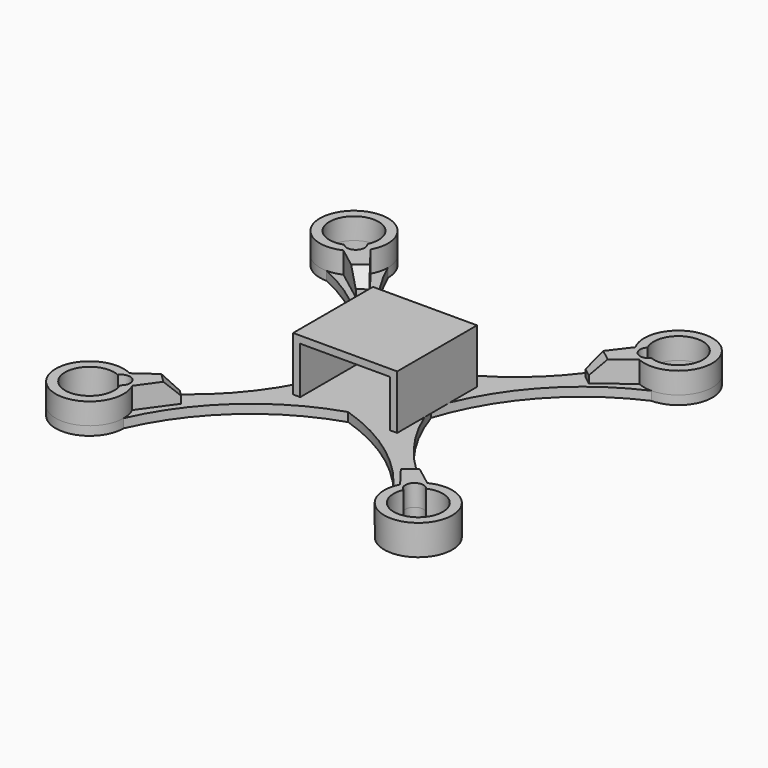
from build123d import *
from build123d import SkipClean  # not in build123d's __all__

# Parameters (mm, degrees)
F0_R     = 3.45
F1_DEPTH = 1.25
F2_R     = 1.27
F3_DEPTH = 15.24
F5_DEPTH = 7
F6_R     = 1.5
F7_DEPTH = 1.25
F9_DEPTH = 3
F10_SIZE = 2


# Not quite as in the source:
# - a feature of the source that left no trace in its solid (it failed there, or was rolled back) is left out


with BuildPart() as f1:
    # F0 (on Top) → F1 (new body)
    with BuildSketch(Plane.XY):
        with BuildLine():
            ThreePointArc((0, 6.477), (-10.7423411653, 12.8214445823), (-17.975, 22.987))
            ThreePointArc((-17.975, 22.987), (-26.1154007446, 26.3744330736), (-22.7811582525, 18.2121016594))
            ThreePointArc((-22.7811582525, 18.2121016594), (-12.6900771407, 10.8419183213), (-6.477, 0))
            ThreePointArc((-6.477, 0), (-12.7950799481, -10.8797937043), (-23.0188417475, -18.2121016594))
            ThreePointArc((-23.0188417475, -18.2121016594), (-26.4374330736, -26.3524007446), (-18.275, -22.987))
            ThreePointArc((-18.275, -22.987), (-10.9098200432, -12.770210249), (0, -6.477))
            ThreePointArc((0, -6.477), (10.9098200432, -12.770210249), (18.275, -22.987))
            ThreePointArc((18.275, -22.987), (26.4374330736, -26.3524007446), (23.0188417475, -18.2121016594))
            ThreePointArc((23.0188417475, -18.2121016594), (12.7950799481, -10.8797937043), (6.477, 0))
            ThreePointArc((6.477, 0), (12.6900771407, 10.8419183213), (22.7811582525, 18.2121016594))
            ThreePointArc((22.7811582525, 18.2121016594), (26.1154007446, 26.3744330736), (17.975, 22.987))
            ThreePointArc((17.975, 22.987), (10.7423411653, 12.8214445823), (0, 6.477))
        make_face()
        with Locations((-23.05, -22.987)):
            Circle(F0_R, mode=Mode.SUBTRACT)
        with Locations((23.05, -22.987)):
            Circle(F0_R, mode=Mode.SUBTRACT)
        with Locations((-22.75, 22.987)):
            Circle(F0_R, mode=Mode.SUBTRACT)
        with Locations((22.75, 22.987)):
            Circle(F0_R, mode=Mode.SUBTRACT)
    extrude(amount=F1_DEPTH)

    # F2 (on face) → F3 (cut)
    with BuildSketch(Plane.XY.offset(1.25)):
        with Locations((-20.5791849834, 20.5791849834)):
            Circle(F2_R)
        with Locations((20.5791849834, 20.5791849834)):
            Circle(F2_R)
        with Locations((20.5791849834, -20.5791849834)):
            Circle(F2_R)
        with Locations((-20.5791849834, -20.5791849834)):
            Circle(F2_R)
    extrude(amount=-F3_DEPTH, mode=Mode.SUBTRACT)

    # F4 (on Front) → F5 (join, symmetric)
    with BuildSketch(Plane.XZ):
        Polygon((-6.3, 1.25), (-6.3, 7.85), (6.3, 7.85), (6.3, 1.25), (7.3, 1.25), (7.3, 8.85), (-7.3, 8.85), (-7.3, 1.25), align=None)
    extrude(amount=F5_DEPTH, both=True)

    # F6 (on face) → F7 (cut, through all)
    with BuildSketch(Plane.XY.offset(1.25)):
        with Locations((0, 6.477)):
            Circle(F6_R)
    extrude(amount=-F7_DEPTH, mode=Mode.SUBTRACT)

    # F8 (on face) → F9 (join)
    with BuildSketch(Plane.XY.offset(1.25)):
        with BuildLine():
            Line((-16.3602319323, -15.5348950992), (-20.8478584952, -18.7501146118))
            ThreePointArc((-20.8478584952, -18.7501146118), (-26.4716233511, -26.3176333696), (-18.7553139698, -20.8998256177))
            Line((-18.7553139698, -20.8998256177), (-15.5117037948, -16.3834232366))
            Line((-15.5117037948, -16.3834232366), (-16.3602319323, -15.5348950992))
        make_face()
        with BuildLine():
            ThreePointArc((-19.8753821862, -21.6363328551), (-25.5208150166, -25.3948150166), (-21.6178063096, -19.8483185518))
            ThreePointArc((-21.6178063096, -19.8483185518), (-19.669638586, -19.6928298904), (-19.8753821862, -21.6363328551))
        make_face(mode=Mode.SUBTRACT)
        with BuildLine():
            Line((15.3199540065, -16.3082468694), (18.7838269987, -20.8421473423))
            ThreePointArc((18.7838269987, -20.8421473423), (26.4264348802, -26.3634348802), (20.9051473423, -18.7208269987))
            Line((20.9051473423, -18.7208269987), (16.5119000472, -15.3976071843))
            Line((16.5119000472, -15.3976071843), (15.3199540065, -16.3082468694))
        make_face()
        with BuildLine():
            ThreePointArc((21.6178063096, -19.8483185518), (25.5208150166, -25.3948150166), (19.8753821862, -21.6363328551))
            ThreePointArc((19.8753821862, -21.6363328551), (19.669638586, -19.6928298904), (21.6178063096, -19.8483185518))
        make_face(mode=Mode.SUBTRACT)
        with BuildLine():
            Line((16.3457305073, 15.2946304795), (20.7653185529, 18.6439982094))
            ThreePointArc((20.7653185529, 18.6439982094), (25.9985065626, 26.4866900024), (18.5665604362, 20.6849447408))
            Line((18.5665604362, 20.6849447408), (15.1525434236, 16.2036434514))
            Line((15.1525434236, 16.2036434514), (16.3457305073, 15.2946304795))
        make_face()
        with BuildLine():
            ThreePointArc((19.659038987, 21.4545313979), (25.0601507831, 25.5493628469), (21.5448562878, 19.7543341291))
            ThreePointArc((21.5448562878, 19.7543341291), (19.7287816517, 19.6359383702), (19.659038987, 21.4545313979))
        make_face(mode=Mode.SUBTRACT)
        with BuildLine():
            ThreePointArc((-18.5665604362, 20.6849447408), (-25.9985065626, 26.4866900024), (-20.7653185529, 18.6439982094))
            Line((-20.7653185529, 18.6439982094), (-16.3523570468, 15.30128828))
            Line((-16.3523570468, 15.30128828), (-15.1589701598, 16.2100389266))
            Line((-15.1589701598, 16.2100389266), (-18.5665604362, 20.6849447408))
        make_face()
        with BuildLine():
            ThreePointArc((-21.5448562878, 19.7543341291), (-25.0601507831, 25.5493628469), (-19.659038987, 21.4545313979))
            ThreePointArc((-19.659038987, 21.4545313979), (-19.3094528761, 20.6052689951), (-19.6238661036, 19.7423661036))
            ThreePointArc((-19.6238661036, 19.7423661036), (-20.5870970996, 19.30920963), (-21.5448562878, 19.7543341291))
        make_face(mode=Mode.SUBTRACT)
    with SkipClean():  # cleaning this boolean's faces spoils the solid; the shape is the same uncleaned
        extrude(amount=F9_DEPTH)

    # F10
    f10_edges = [f1.edges().sort_by_distance(p)[0] for p in [
        (-15.755664, 15.755664, 4.25),
        (-15.935968, -15.959159, 4.25),
        (15.915927, -15.852927, 4.25),
        (15.749137, 15.749137, 4.25),
    ]]
    chamfer(f10_edges, length=F10_SIZE)


solid = f1.part
